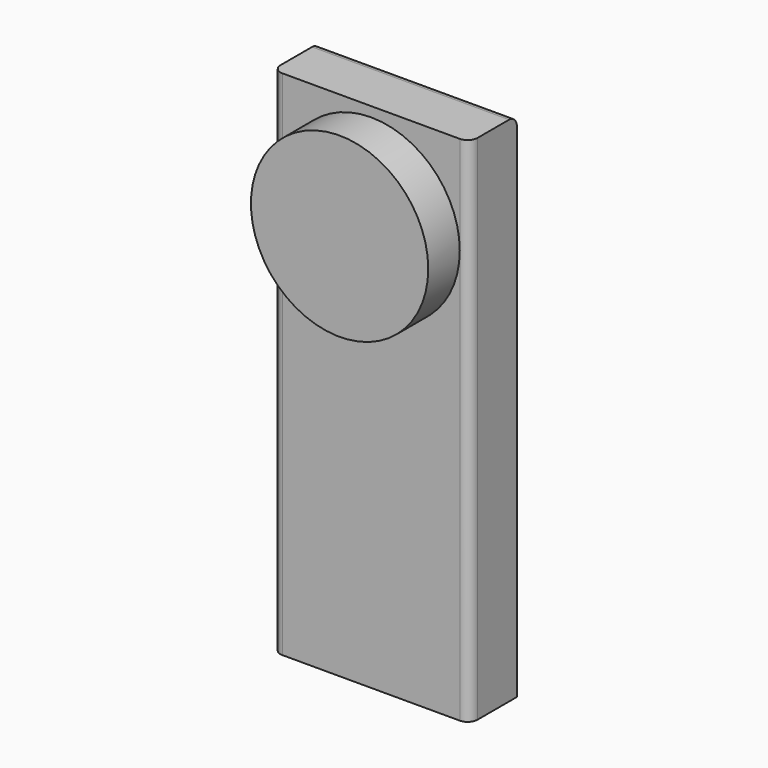
from build123d import *

# Parameters (mm, degrees)
F0_W        = 100
F0_H        = 260
F1_DEPTH    = 30
F3_R        = 5
F2_R        = 45
F4_DEPTH    = 20
F5_T        = 5
F5_T4_ANGLE = 180.000000001
F5_T6_ANGLE = 180.000000001


# Not quite as in the source:
# - a shell that OpenCascade refuses in one call is made with other operations: the cavity is built on its own and cut out


with BuildPart() as f1:
    # F0 (on Front) → F1 (new body)
    with BuildSketch(Plane.XZ):
        with Locations((-0.186801888, -30)):
            Rectangle(F0_W, F0_H)
    extrude(amount=-F1_DEPTH)

    # F3
    f3_edges = [f1.edges().sort_by_distance(p)[0] for p in [
        (49.813198, 0, -30),
        (-50.186802, 0, -30),
        (-0.186802, 30, 100),
    ]]
    fillet(f3_edges, radius=F3_R)

    # F2 (on Front) → F4 (join)
    with BuildSketch(Plane.XZ):
        with Locations((-0.186801888, 50)):
            Circle(F2_R)
    extrude(amount=F4_DEPTH)

    # F5: shell of thickness 5, made by hand


with BuildPart() as f5_core1:
    # F5_t2: copy of F1
    add(f1.part)

    # the walls: a layer under each face that stays
    f5_faces = [f5_core1.faces().sort_by_distance(p)[0] for p in [
        (-0.186801888, 12.5, 100),
        (49.813198112, 17.5, -30),
        (-30.186801888, 0, 91.6666666667),
        (-50.186801888, 17.5, -30),
        (-0.186801888, 30, -32.5),
        (-0.186801888, 0, -55),
        (-45.186801888, -10, 50),
        (-0.186801888, -20, 50),
    ]]
    thicken(f5_faces, amount=-F5_T, mode=Mode.SUBTRACT)

    # F5_s3 → F5_t4 (revolve, cut)
    with BuildSketch(Plane.XY.offset(50)):
        Polygon((44.863198112, -0.05), (44.813198112, 5), (39.813198112, 5), (39.813198112, 0), align=None)
    revolve(axis=Axis((-0.186801888, 0, 50), (0, -1, 0)), revolution_arc=F5_T4_ANGLE, mode=Mode.SUBTRACT)

    # F5_s5 → F5_t6 (revolve, cut)
    with BuildSketch(Plane.XY.offset(50)):
        Polygon((-45.236801888, -0.05), (-45.186801888, 5), (-40.186801888, 5), (-40.186801888, 0), align=None)
    revolve(axis=Axis((-0.186801888, 0, 50), (0, -1, 0)), revolution_arc=F5_T6_ANGLE, mode=Mode.SUBTRACT)


with BuildPart() as f1_1:
    add(f1.part)

    # what is left inside the walls is the cavity
    f5_cavity = [f5_core1.part.solids().sort_by_distance(p)[0] for p in [
        (-0.186802, 24.95, -75),
    ]]
    add(f5_cavity, mode=Mode.SUBTRACT)


solid = f1_1.part
